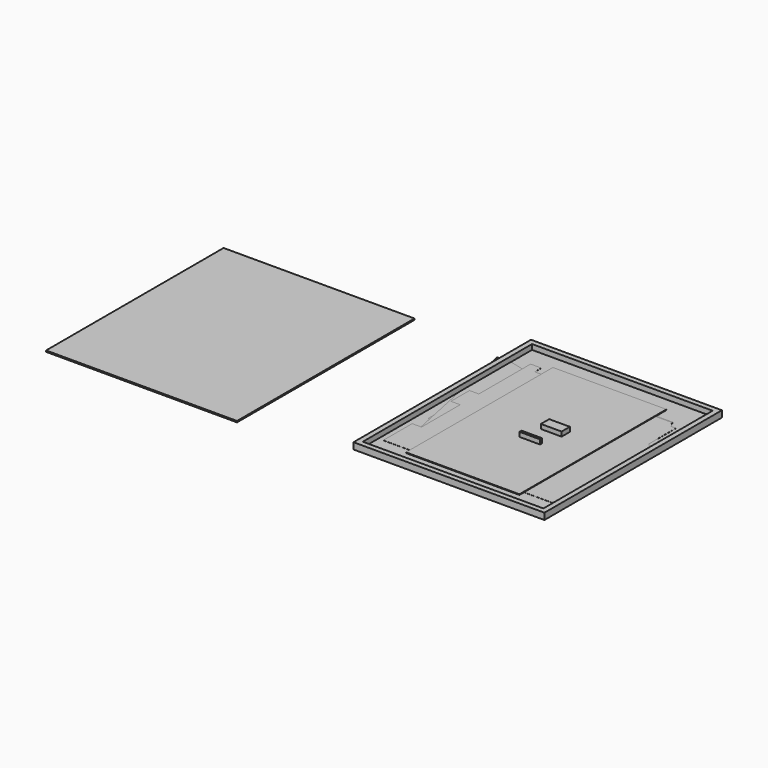
from build123d import *

# Parameters (mm, degrees)
F1_DEPTH  = 0.508
F2_R      = 2.54
F4_DEPTH  = 0.508
F5_R      = 2.54
F6_R      = 50.8
F8_DEPTH  = 0.508
F9_R      = 2.54
F10_W     = 939.8
F10_H     = 1092.2
F10_W_2   = 889
F10_H_2   = 1041.4
F11_DEPTH = 25.4
F12_DEPTH = 6.35
F15_W     = 101.6
F15_H     = 50.8
F16_DEPTH = 25.4
F17_W     = 101.6
F17_H     = 12.7
F18_DEPTH = 25.4
F19_W     = 558.8
F19_H     = 904.494
F20_DEPTH = 0.508
F21_DEPTH = 2.54
F22_DEPTH = 3.175
F23_DEPTH = 2.54
F24_W     = 939.8
F24_H     = 1092.2
F25_DEPTH = 6.35


with BuildPart() as f1:
    # F0 (on Top) → F1 (new body)
    with BuildSketch(Plane.XY):
        Polygon((230.6246389754, 290.787051339), (-243.3404602368, 292.064576269), (-243.3404602368, 202.1270656108), (-457.9661569358, 202.1270656108), (-457.9661569358, 99.9243696019), (-399.1995891905, 99.9243696019), (-399.1995891905, -176.0229797828), (-243.3404602368, -176.0229797828), (-243.3404602368, -268.005423731), (230.6246389754, -268.005423731), (230.6246389754, -178.0679043027), (346.8802319958, -178.0679043027), (381.3736155884, -212.5613317459), (446.5278430642, -212.5613317459), (446.5278430642, -145.3621622101), (401.8141547902, -67.432584578), (401.8141547902, 88.4265575308), (446.5278430642, 167.6336644779), (446.5278430642, 237.8980442943), (380.0961257389, 237.8980442943), (346.8802319958, 202.1270656108), (230.6246389754, 202.1270656108), align=None)
    extrude(amount=F1_DEPTH)

    # F2
    f2_edges = [f1.edges().sort_by_distance(p)[0] for p in [
        (-243.34046, 292.064576, 0.254),
        (-243.34046, 202.127066, 0.254),
        (-457.966157, 202.127066, 0.254),
        (-457.966157, 99.92437, 0.254),
        (-399.199589, 99.92437, 0.254),
        (-399.199589, -176.02298, 0.254),
        (-243.34046, -176.02298, 0.254),
        (-243.34046, -268.005424, 0.254),
        (230.624639, -268.005424, 0.254),
        (230.624639, -178.067904, 0.254),
        (381.373616, -212.561332, 0.254),
        (446.527843, -212.561332, 0.254),
        (446.527843, 237.898044, 0.254),
        (380.096126, 237.898044, 0.254),
        (230.624639, 202.127066, 0.254),
        (230.624639, 290.787051, 0.254),
    ]]
    fillet(f2_edges, radius=F2_R)


with BuildPart() as f4:
    # F3 (on Top) → F4 (new body)
    with BuildSketch(Plane.XY):
        Polygon((-433.5246007602, 387.6472785744), (-510.2978141339, 388.9824003828), (-354.8711431147, -350.9195996172), (-158.2375419669, -350.9195996172), (-158.2375419669, -218.6388209421), (0, -218.6388209421), (0, -348.8350246486), (199.2781225235, -348.8350246486), (360.1601858661, 387.6472785744), (277.9315944909, 387.6472785744), (-77.7965102956, 300.0559436386), align=None)
    extrude(amount=F4_DEPTH)

    # F5
    f5_edges = [f4.edges().sort_by_distance(p)[0] for p in [
        (-158.237542, -350.9196, 0.254),
        (-158.237542, -218.638821, 0.254),
        (0, -218.638821, 0.254),
        (0, -348.835025, 0.254),
        (-354.871143, -350.9196, 0.254),
        (199.278123, -348.835025, 0.254),
        (360.160186, 387.647279, 0.254),
        (-510.297814, 388.9824, 0.254),
    ]]
    fillet(f5_edges, radius=F5_R)

    # F6
    f6_edges = [f4.edges().sort_by_distance(p)[0] for p in [
        (-77.79651, 300.055944, 0.254),
    ]]
    fillet(f6_edges, radius=F6_R)


with BuildPart() as f8:
    # F7 (on Top) → F8 (new body)
    with BuildSketch(Plane.XY):
        Polygon((-321.2298876628, 424.3650341868), (-374.287745627, 424.3650341868), (-374.287745627, 105.567770452), (-420.1756300418, 105.567770452), (-420.1756300418, -9.1519531711), (-374.287745627, -9.1519531711), (-374.287745627, -247.1953801433), (-420.1756300418, -247.1953801433), (-420.1756300418, -425.0109658132), (421.5803699582, -425.0109658132), (421.5803699582, 164.3616363428), (395.7684293811, 188.739577735), (395.7684293811, 356.5171802986), (371.3904656141, 356.5171802986), (354.1825201459, 383.7630976857), (248.066759468, 383.7630976857), (229.424814815, 353.649181929), (-186.434210413, 353.649181929), (-205.076155066, 383.7630976857), (-321.2298876628, 383.7630976857), align=None)
    extrude(amount=F8_DEPTH)

    # F9
    f9_edges = [f8.edges().sort_by_distance(p)[0] for p in [
        (-374.287746, 424.365034, 0.254),
        (-374.287746, 105.56777, 0.254),
        (-420.17563, 105.56777, 0.254),
        (-420.17563, -9.151953, 0.254),
        (-374.287746, -9.151953, 0.254),
        (-374.287746, -247.19538, 0.254),
        (-420.17563, -247.19538, 0.254),
        (-420.17563, -425.010966, 0.254),
        (421.58037, -425.010966, 0.254),
        (395.768429, 356.51718, 0.254),
        (354.18252, 383.763098, 0.254),
        (248.066759, 383.763098, 0.254),
        (-205.076155, 383.763098, 0.254),
        (-321.229888, 383.763098, 0.254),
        (-321.229888, 424.365034, 0.254),
    ]]
    fillet(f9_edges, radius=F9_R)


with BuildPart() as f11:
    # F10 (on Top) → F11 (new body)
    with BuildSketch(Plane.XY):
        Rectangle(F10_W, F10_H)
        Rectangle(F10_W_2, F10_H_2, mode=Mode.SUBTRACT)
    extrude(amount=F11_DEPTH)

    # F10 (on Top) → F12 (join)
    with BuildSketch(Plane.XY):
        Rectangle(F10_W, F10_H)
        Rectangle(F10_W_2, F10_H_2, mode=Mode.SUBTRACT)
        Rectangle(F10_W_2, F10_H_2)
    extrude(amount=-F12_DEPTH)


with BuildPart() as f16:
    # F15 (on Top) → F16 (new body)
    with BuildSketch(Plane.XY):
        with Locations((48.4836730175, 48.1311040878)):
            Rectangle(F15_W, F15_H)
    extrude(amount=F16_DEPTH)


with BuildPart() as f18:
    # F17 (on Top) → F18 (new body)
    with BuildSketch(Plane.XY):
        with Locations((25.0777602196, -73.6970956956)):
            Rectangle(F17_W, F17_H)
    extrude(amount=F18_DEPTH)


with BuildPart() as f20:
    # F19 (on Top) → F20 (new body)
    with BuildSketch(Plane.XY):
        with Locations((-7.2680772661, -0.4515498877)):
            Rectangle(F19_W, F19_H)
    extrude(amount=F20_DEPTH)


with BuildPart() as f21:
    # F19 (on Top) → F21 (new body)
    with BuildSketch(Plane.XY):
        with Locations((-7.2680772661, -0.4515498877)):
            Rectangle(F19_W, F19_H)
    extrude(amount=F21_DEPTH)


with BuildPart() as f22:
    # F19 (on Top) → F22 (new body)
    with BuildSketch(Plane.XY):
        with Locations((-7.2680772661, -0.4515498877)):
            Rectangle(F19_W, F19_H)
    extrude(amount=F22_DEPTH)


with BuildPart() as f23:
    # F19 (on Top) → F23 (new body)
    with BuildSketch(Plane.XY):
        with Locations((-7.2680772661, -0.4515498877)):
            Rectangle(F19_W, F19_H)
    extrude(amount=F23_DEPTH)


with BuildPart() as f25:
    # F24 (on Top) → F25 (new body)
    with BuildSketch(Plane.XY):
        with Locations((-1422.8657513078, -113.0663752556)):
            Rectangle(F24_W, F24_H)
    extrude(amount=F25_DEPTH)


solid = Compound([f1.part, f4.part, f8.part, f11.part, f16.part, f18.part, f20.part, f21.part, f22.part, f23.part, f25.part])
